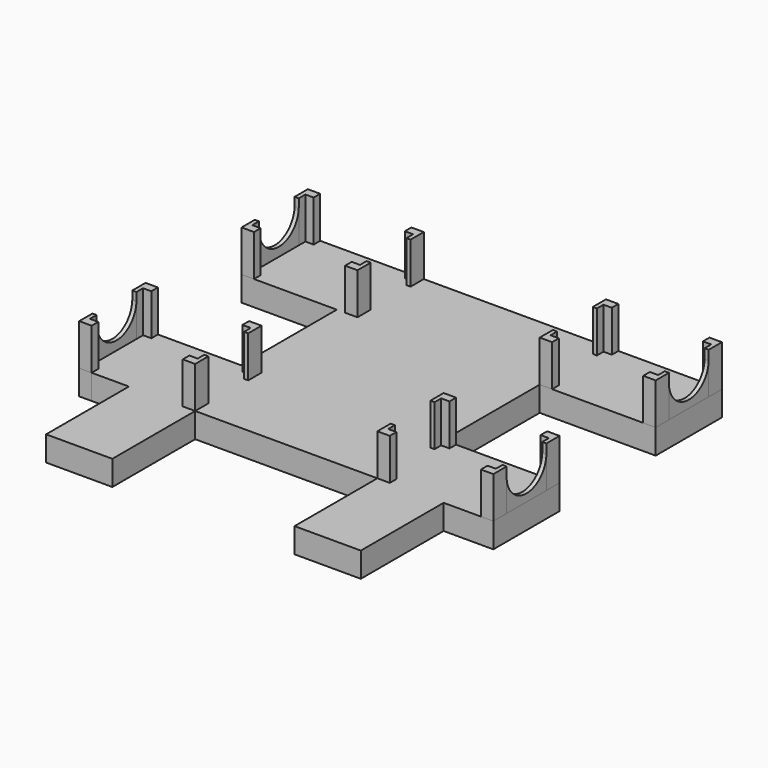
from build123d import *
from build123d import SkipClean  # not in build123d's __all__

# Parameters (mm, degrees)
F1_DEPTH  = 6
F3_DEPTH  = 10
F5_DEPTH  = 1
F7_DEPTH  = 1
F9_DEPTH  = 1
F10_DEPTH = 1
F13_DEPTH = 1


# Not quite as in the source:
# - ends of sketch curves that miss each other by under 0.0002 mm in the source are joined


with BuildPart() as f1:
    # F0 (on Top) → F1 (new body)
    with BuildSketch(Plane.XY):
        Polygon((-60, -8.2803227458), (-60, -33.2803227458), (-44, -33.2803227458), (-44, -8.2803227458), (0, -8.2803227458), (0, -33.2803227458), (16, -33.2803227458), (16, -8.2803227458), (28, -8.2803227458), (28, 11.7196772542), (0, 11.7196772542), (0, 40.7196772542), (28, 40.7196772542), (28, 60.7196772542), (-72, 60.7196772542), (-72, 40.7196772542), (-49, 40.7196772542), (-49, 11.7196772542), (-72, 11.7391310632), (-72, 11.693589665), (-72, 7.693589665), (-72, -4.280322887), (-72, -8.280322887), (-69, -8.2803227458), align=None)
    extrude(amount=F1_DEPTH)

    # F2 (on face) → F3 (join)
    with BuildSketch(Plane.XY.offset(6)):
        Polygon((-72, 60.7196772542), (-72, 56.7391310632), (-71, 56.7391310632), (-71, 58.7391310632), (-69, 58.7391310632), (-69, 60.7196772542), align=None)
        Polygon((-72, 40.7196773953), (-69, 40.7196773953), (-69, 42.7196773953), (-71, 42.7196773953), (-71, 44.7196773953), (-72, 44.7196773953), align=None)
        Polygon((-45, 42.7196773953), (-47, 42.7196773953), (-47, 40.7196773953), (-44, 40.7196773953), (-44, 44.7196773953), (-45, 44.7196773953), align=None)
        Polygon((-44, 60.7196772542), (-47, 60.7196772542), (-47, 58.7391310632), (-45, 58.7391310632), (-45, 56.7391310632), (-44, 56.7391310632), align=None)
        Polygon((28, 60.7196772542), (25, 60.7196772542), (25, 58.7391310632), (27, 58.7391310632), (27, 56.7391310632), (28, 56.7391310632), align=None)
        Polygon((25, 42.7196773953), (25, 40.7196773953), (28, 40.7196773953), (28, 44.7196773953), (27, 44.7196773953), (27, 42.7196773953), align=None)
        Polygon((0, 44.7196773953), (0, 40.7196772542), (3, 40.7196773953), (3, 42.7196773953), (1, 42.7196773953), (1, 44.7196773953), align=None)
        Polygon((3, 60.7196772542), (0, 60.7196772542), (0, 56.7391310632), (1, 56.7391310632), (1, 58.7391310632), (3, 58.7391310632), align=None)
        Polygon((27, 7.7391309221), (28, 7.7391309221), (28, 11.7196772542), (25, 11.7196772542), (25, 9.7391309221), (27, 9.7391309221), align=None)
        Polygon((25, -6.2803227458), (25, -8.2803227458), (28, -8.2803227458), (28, -4.2803227458), (27, -4.2803227458), (27, -6.2803227458), align=None)
        Polygon((0, -4.2803227458), (0, -8.280322887), (3, -8.2803227458), (3, -6.2803227458), (1, -6.2803227458), (1, -4.2803227458), align=None)
        Polygon((3, 9.7391309221), (3, 11.7196772542), (0, 11.7196772542), (0, 7.7391309221), (1, 7.7391309221), (1, 9.7391309221), align=None)
        Polygon((-45, 7.7391309221), (-44, 7.7391309221), (-44, 11.7391310632), (-47, 11.7391309221), (-47, 9.7391309221), (-45, 9.7391309221), align=None)
        Polygon((-47, -8.2803227458), (-44, -8.2803227458), (-44, -4.2803227458), (-45, -4.2803227458), (-45, -6.2803227458), (-47, -6.2803227458), align=None)
        Polygon((-72, -4.2803227458), (-72, -8.280322887), (-69, -8.2803227458), (-69, -6.2803227458), (-71, -6.2803227458), (-71, -4.2803227458), align=None)
        Polygon((-72, 11.7391310632), (-72, 7.7391309221), (-71, 7.7391309221), (-71, 9.7391309221), (-69, 9.7391309221), (-69, 11.7365936099), align=None)
    with SkipClean():  # cleaning this boolean's faces spoils the solid; the shape is the same uncleaned
        extrude(amount=F3_DEPTH)

    # F4 (on face) → F5 (join)
    with BuildSketch(Plane.YZ.offset(28)):
        with BuildLine():
            ThreePointArc((7.7391309221, 13.6681435205), (1.7294040881, 7.8220547277), (-4.2803227458, 13.6681435205))
            Line((-4.2803227458, 13.6681435205), (-4.2803227458, 6))
            Line((-4.2803227458, 6), (7.7391309221, 6))
            Line((7.7391309221, 6), (7.7391309221, 13.6681435205))
        make_face()
    with SkipClean():  # cleaning this boolean's faces spoils the solid; the shape is the same uncleaned
        extrude(amount=-F5_DEPTH)

    # F6 (on face) → F7 (join)
    with BuildSketch(Plane.YZ.offset(28)):
        with BuildLine():
            ThreePointArc((56.7391310632, 13.6693800888), (50.7294042293, 7.8226900444), (44.7196773953, 13.6693800888))
            Line((44.7196773953, 13.6693800888), (44.7196773953, 6))
            Line((44.7196773953, 6), (56.7391310632, 6))
            Line((56.7391310632, 6), (56.7391310632, 13.6693800888))
        make_face()
    with SkipClean():  # cleaning this boolean's faces spoils the solid; the shape is the same uncleaned
        extrude(amount=-F7_DEPTH)

    # F8 (on face) → F9 (join)
    with BuildSketch(Plane(origin=(-72, 0, 0), x_dir=(0, -1, 0), z_dir=(-1, 0, 0))):
        with BuildLine():
            ThreePointArc((-44.7196773953, 14), (-50.7294042293, 8.1363701718), (-56.7391310632, 14))
            Line((-56.7391310632, 14), (-56.7391310632, 6))
            Line((-56.7391310632, 6), (-44.7196773953, 6))
            Line((-44.7196773953, 6), (-44.7196773953, 14))
        make_face()
    with SkipClean():  # cleaning this boolean's faces spoils the solid; the shape is the same uncleaned
        extrude(amount=-F9_DEPTH)

    # F12 (on face) → F13 (join)
    with BuildSketch(Plane(origin=(-72, 0, 0), x_dir=(0, -1, 0), z_dir=(-1, 0, 0))):
        with BuildLine():
            ThreePointArc((4.2803227458, 14), (-1.7294040881, 8.1533099556), (-7.7391309221, 14))
            Line((-7.7391309221, 14), (-7.7391309221, 6))
            Line((-7.7391309221, 6), (4.2803227458, 6))
            Line((4.2803227458, 6), (4.2803227458, 14))
        make_face()
    with SkipClean():  # cleaning this boolean's faces spoils the solid; the shape is the same uncleaned
        extrude(amount=-F13_DEPTH)


with BuildPart() as f10:
    # F8 (on face) → F10 (new body)
    with BuildSketch(Plane(origin=(-72, 0, 0), x_dir=(0, -1, 0), z_dir=(-1, 0, 0))):
        with BuildLine():
            ThreePointArc((4.282593064, 13.8288382557), (-1.649666924, 7.8232188447), (-7.7391309221, 13.6693800888))
            Line((-7.7391309221, 13.6693800888), (-7.7391309221, 5.9489118867))
            Line((-7.7391309221, 5.9489118867), (4.3871137314, 5.9489118867))
            Line((4.3871137314, 5.9489118867), (4.282593064, 13.8288382557))
        make_face()
    extrude(amount=-F10_DEPTH)


solid = f1.part
